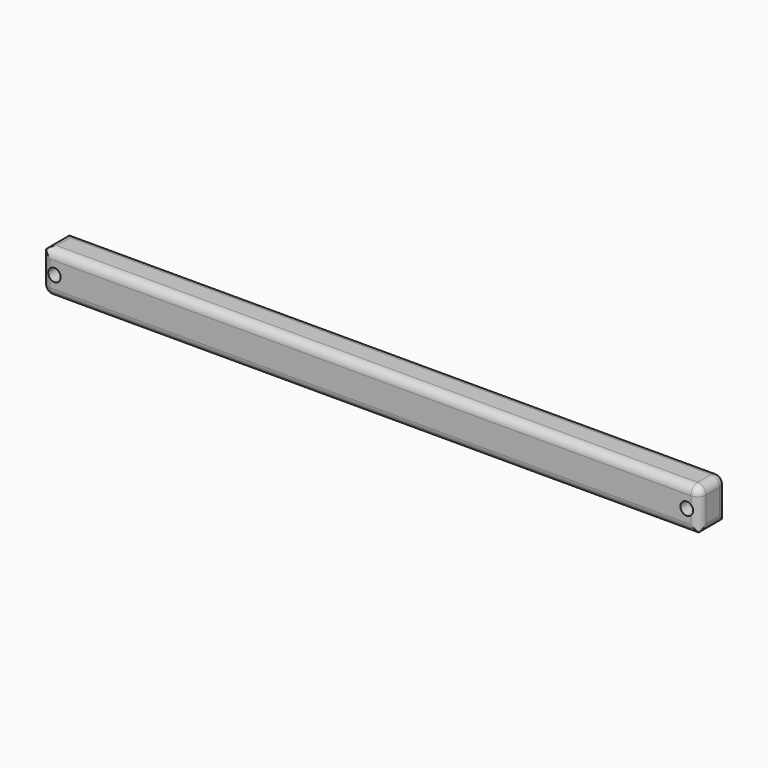
from build123d import *

# Parameters (mm, degrees)
F0_W         = 156
F0_H         = 10
F0_R         = 1.5
F1_DEPTH     = 8
F2_T1_DEPTH  = 4
F2_T3_DEPTH  = 18
F2_T5_DEPTH  = 159
F2_T7_DEPTH  = 13
F2_S11_W     = 2
F2_S11_H     = 2
F2_T12_DEPTH = 2
F2_S17_W     = 2
F2_S17_H     = 2
F2_T18_DEPTH = 2
F3_T1_DEPTH  = 11
F3_T3_DEPTH  = 4
F3_T5_DEPTH  = 157
F3_S9_W      = 2.04
F3_S9_H      = 2.04
F3_T10_DEPTH = 2.04
F3_S15_W     = 2.04
F3_S15_H     = 2.04
F3_T16_DEPTH = 2.04


# Not quite as in the source:
# - a fillet or chamfer that OpenCascade refuses, or shapes differently, is made with other operations: its cross-section is extruded or revolved along the edge and cut away or added


with BuildPart() as f1:
    # F0 (on Front) → F1 (new body)
    with BuildSketch(Plane.XZ):
        with Locations((-25, 5)):
            Rectangle(F0_W, F0_H)
        with Locations((-100, 5)):
            Circle(F0_R, mode=Mode.SUBTRACT)
        with Locations((50, 5)):
            Circle(F0_R, mode=Mode.SUBTRACT)
    extrude(amount=F1_DEPTH)

    # F2: fillet of radius 2 on 7 edges, made by hand

    # F2_s2 → F2_t1 (cut)
    with BuildSketch(Plane.XZ.offset(2)):
        with BuildLine():
            ThreePointArc((53, 8), (52.4142135624, 9.4142135624), (51, 10))
            Line((51, 10), (53, 10))
            Line((53, 10), (53, 8))
        make_face()
    extrude(amount=F2_T1_DEPTH, mode=Mode.SUBTRACT)

    # F2_s4 → F2_t3 (cut)
    with BuildSketch(Plane.XZ.offset(-5)):
        with BuildLine():
            ThreePointArc((-103, 8), (-102.4142135624, 9.4142135624), (-101, 10))
            Line((-101, 10), (-103, 10))
            Line((-103, 10), (-103, 8))
        make_face()
        with BuildLine():
            ThreePointArc((51, 0), (52.4142135624, 0.5857864376), (53, 2))
            Line((53, 2), (53, 0))
            Line((53, 0), (51, 0))
        make_face()
    extrude(amount=F2_T3_DEPTH, mode=Mode.SUBTRACT)

    # F2_s6 → F2_t5 (cut)
    with BuildSketch(Plane.YZ.offset(-108)):
        with BuildLine():
            ThreePointArc((-2, 10), (-0.5857864376, 9.4142135624), (0, 8))
            Line((0, 8), (0, 10))
            Line((0, 10), (-2, 10))
        make_face()
        with BuildLine():
            ThreePointArc((-6, 10), (-7.4142135624, 9.4142135624), (-8, 8))
            Line((-8, 8), (-8, 10))
            Line((-8, 10), (-6, 10))
        make_face()
    extrude(amount=F2_T5_DEPTH, mode=Mode.SUBTRACT)

    # F2_s8 → F2_t7 (cut)
    with BuildSketch(Plane.XY.offset(-5)):
        with BuildLine():
            ThreePointArc((53, -2), (52.4142135624, -0.5857864376), (51, 0))
            Line((51, 0), (53, 0))
            Line((53, 0), (53, -2))
        make_face()
        with BuildLine():
            ThreePointArc((53, -6), (52.4142135624, -7.4142135624), (51, -8))
            Line((51, -8), (53, -8))
            Line((53, -8), (53, -6))
        make_face()
    extrude(amount=F2_T7_DEPTH, mode=Mode.SUBTRACT)


with BuildPart() as f2_tool10:
    # F2_s11 → F2_t12 (new body)
    with BuildSketch(Plane.YZ.offset(51)):
        with Locations((-1, 9)):
            Rectangle(F2_S11_W, F2_S11_H)
    extrude(amount=F2_T12_DEPTH)

    # F2_s13 → F2_t14 (revolve, cut)
    with BuildSketch(Plane(origin=(51, -2, 8), x_dir=(0, -0.7071067812, -0.7071067812), z_dir=(0, -0.7071067812, 0.7071067812))):
        with BuildLine():
            ThreePointArc((0, -2), (2, 0), (0, 2))
            Line((0, 2), (0, -2))
        make_face()
    revolve(axis=Axis((51, -2, 8), (1, 0, 0)), mode=Mode.SUBTRACT)


with BuildPart() as f1_1:
    add(f1.part)

    # F2_t9: cut F2_tool10
    add(f2_tool10.part, mode=Mode.SUBTRACT)


with BuildPart() as f2_tool16:
    # F2_s17 → F2_t18 (new body)
    with BuildSketch(Plane.YZ.offset(51)):
        with Locations((-7, 9)):
            Rectangle(F2_S17_W, F2_S17_H)
    extrude(amount=F2_T18_DEPTH)

    # F2_s19 → F2_t20 (revolve, cut)
    with BuildSketch(Plane(origin=(51, -6, 8), x_dir=(0, 0.7071067812, -0.7071067812), z_dir=(0, -0.7071067812, -0.7071067812))):
        with BuildLine():
            ThreePointArc((0, -2), (2, 0), (0, 2))
            Line((0, 2), (0, -2))
        make_face()
    revolve(axis=Axis((51, -6, 8), (1, 0, 0)), mode=Mode.SUBTRACT)


with BuildPart() as f1_2:
    add(f1_1.part)

    # F2_t15: cut F2_tool16
    add(f2_tool16.part, mode=Mode.SUBTRACT)

    # F3: fillet of radius 2 on 7 edges, made by hand

    # F3_s2 → F3_t1 (cut)
    with BuildSketch(Plane.XY.offset(2)):
        with BuildLine():
            ThreePointArc((-103, -2), (-102.4142135624, -0.5857864376), (-101, 0))
            Line((-101, 0), (-103, 0))
            Line((-103, 0), (-103, -2))
        make_face()
        with BuildLine():
            ThreePointArc((-103, -6), (-102.4142135624, -7.4142135624), (-101, -8))
            Line((-101, -8), (-103, -8))
            Line((-103, -8), (-103, -6))
        make_face()
    extrude(amount=F3_T1_DEPTH, mode=Mode.SUBTRACT)

    # F3_s4 → F3_t3 (cut)
    with BuildSketch(Plane.XZ.offset(2)):
        with BuildLine():
            ThreePointArc((-103, 2), (-102.4142135624, 0.5857864376), (-101, 0))
            Line((-101, 0), (-103, 0))
            Line((-103, 0), (-103, 2))
        make_face()
    extrude(amount=F3_T3_DEPTH, mode=Mode.SUBTRACT)

    # F3_s6 → F3_t5 (cut)
    with BuildSketch(Plane.YZ.offset(-101)):
        with BuildLine():
            ThreePointArc((0, 2), (-0.5857864376, 0.5857864376), (-2, 0))
            Line((-2, 0), (0, 0))
            Line((0, 0), (0, 2))
        make_face()
        with BuildLine():
            ThreePointArc((-6, 0), (-7.4142135624, 0.5857864376), (-8, 2))
            Line((-8, 2), (-8, 0))
            Line((-8, 0), (-6, 0))
        make_face()
    extrude(amount=F3_T5_DEPTH, mode=Mode.SUBTRACT)


with BuildPart() as f3_tool8:
    # F3_s9 → F3_t10 (new body)
    with BuildSketch(Plane.YZ.offset(-101)):
        with Locations((-0.98, 0.98)):
            Rectangle(F3_S9_W, F3_S9_H)
    extrude(amount=-F3_T10_DEPTH)

    # F3_s11 → F3_t12 (revolve, cut)
    with BuildSketch(Plane(origin=(-101, -2, 2), x_dir=(0, -0.7071067812, 0.7071067812), z_dir=(0, -0.7071067812, -0.7071067812))):
        with BuildLine():
            ThreePointArc((0, -2), (2, 0), (0, 2))
            Line((0, 2), (0, -2))
        make_face()
    revolve(axis=Axis((-101, -2, 2), (-1, 0, 0)), mode=Mode.SUBTRACT)


with BuildPart() as f1_3:
    add(f1_2.part)

    # F3_t7: cut F3_tool8
    add(f3_tool8.part, mode=Mode.SUBTRACT)


with BuildPart() as f3_tool14:
    # F3_s15 → F3_t16 (new body)
    with BuildSketch(Plane.YZ.offset(-101)):
        with Locations((-7.02, 0.98)):
            Rectangle(F3_S15_W, F3_S15_H)
    extrude(amount=-F3_T16_DEPTH)

    # F3_s17 → F3_t18 (revolve, cut)
    with BuildSketch(Plane(origin=(-101, -6, 2), x_dir=(0, 0.7071067812, 0.7071067812), z_dir=(0, -0.7071067812, 0.7071067812))):
        with BuildLine():
            ThreePointArc((0, -2), (2, 0), (0, 2))
            Line((0, 2), (0, -2))
        make_face()
    revolve(axis=Axis((-101, -6, 2), (-1, 0, 0)), mode=Mode.SUBTRACT)


with BuildPart() as f1_4:
    add(f1_3.part)

    # F3_t13: cut F3_tool14
    add(f3_tool14.part, mode=Mode.SUBTRACT)


solid = f1_4.part
